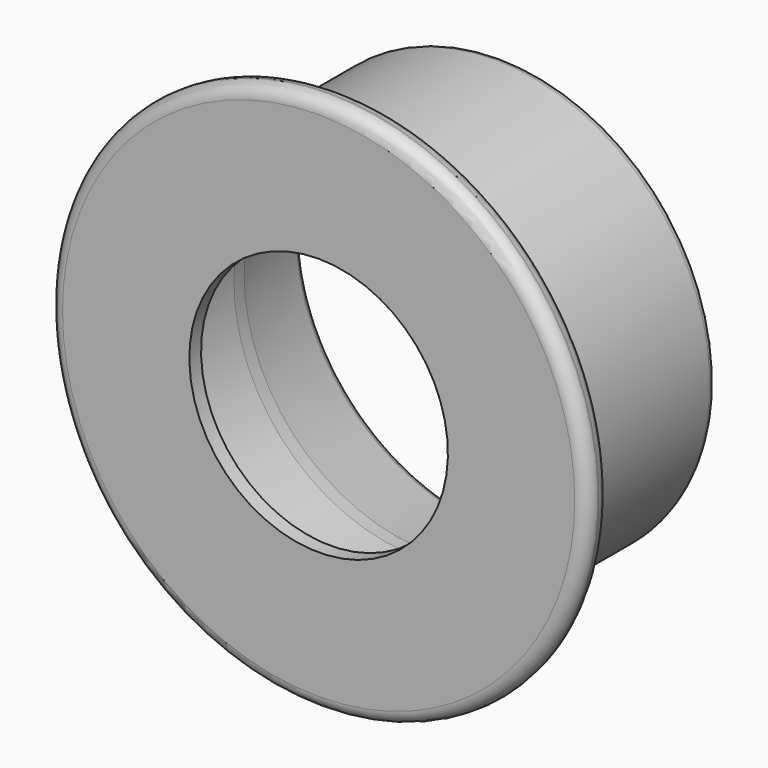
from build123d import *

# Parameters (mm, degrees)
F2_R = 0.8
F3_R = 5


# Not quite as in the source:
# - a feature names something its author has since deleted; it is built from what else it names


with BuildPart() as f1:
    # F0 (on Right) → F1 (revolve)
    with BuildSketch(Plane.YZ):
        Polygon((-3.1, -1), (4, -1), (4, 0), (4, 1), (0, 1), (-4, 1), (-4, -1), align=None)
        Polygon((-3.1, -4.3), (-3.1, -1), (-4, -1), (-4, -2), (-4, -4.3), align=None)
        with BuildLine():
            Line((-4, 3.2), (-4, 1))
            Line((-4, 1), (0, 1))
            add(Edge.make_bspline(
                [(-2.2627416998, 3.2), (-1.6970562748, 1), (0, 1)],
                knots=[5.0522258898, 5.0522258898, 5.0522258898, 6.2831853072, 6.2831853072, 6.2831853072], degree=2, weights=[1, 0.8164965809, 1]))
            Line((-2.2627416998, 3.2), (-4, 3.2))
        make_face()
        with BuildLine():
            Line((-4, 4.3), (-4, 3.2))
            Line((-4, 3.2), (-2.2627416998, 3.2))
            add(Edge.make_bspline(
                [(-2.4, 4.3), (-2.4, 3.7338095117), (-2.2627416998, 3.2)],
                knots=[4.7123889804, 4.7123889804, 4.7123889804, 5.0522258898, 5.0522258898, 5.0522258898], degree=2, weights=[1, 0.9855985597, 1]))
            Line((-2.4, 4.3), (-4, 4.3))
        make_face()
        with BuildLine():
            Line((4, 1), (4, 0))
            Line((4, 0), (9.5, 0))
            ThreePointArc((9.5, 0), (9.1464466094, 0.1464466094), (9, 0.5))
            ThreePointArc((9, 0.5), (9.1464466094, 0.8535533906), (9.5, 1))
            Line((9.5, 1), (4, 1))
        make_face()
        with BuildLine():
            ThreePointArc((9, 0.5), (9.1464466094, 0.1464466094), (9.5, 0))
            ThreePointArc((9.5, 0), (9.5445491992, 0.0019885856), (9.5887440387, 0.0079385246))
            ThreePointArc((9.5887440387, 0.0079385246), (9.883648289, 0.1793537926), (10, 0.5))
            Line((10, 0.5), (9, 0.5))
        make_face()
        with BuildLine():
            ThreePointArc((10, 0.5), (9.8535533906, 0.8535533906), (9.5, 1))
            ThreePointArc((9.5, 1), (9.1464466094, 0.8535533906), (9, 0.5))
            Line((9, 0.5), (10, 0.5))
        make_face()
        Polygon((4, 0), (4, -1), (9.5447270865, 0), (9.5, 0), align=None)
    revolve(axis=Axis((0, 0, -12.25), (0, 1, 0)))

    # F2
    f2_edges = [f1.edges().sort_by_distance(p)[0] for p in [
        (0, -1.822195, 2.152356),
        (0, -2.4, -28.8),
        (0, -4, -28.8),
    ]]
    fillet(f2_edges, radius=F2_R)

    # F3
    f3_edges = [f1.edges().sort_by_distance(p)[0] for p in [
        (0, 4, -23.5),
    ]]
    fillet(f3_edges, radius=F3_R)


solid = f1.part
